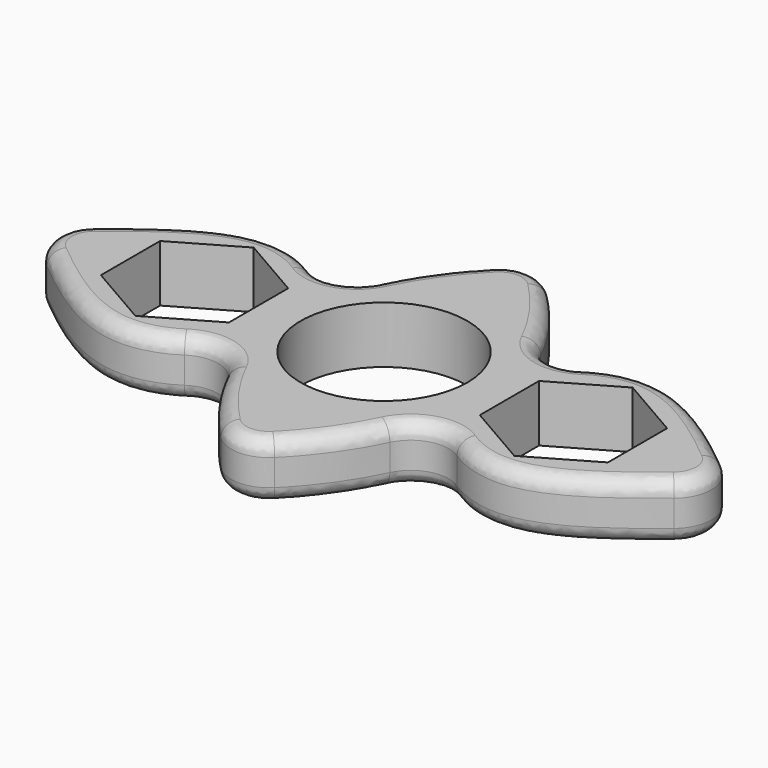
from build123d import *

# Parameters (mm, degrees)
F0_R     = 11
F1_DEPTH = 7.5
F2_R     = 5
F3_R     = 5
F4_R     = 2


# Not quite as in the source:
# - a feature names something its author has since deleted; it is built from what else it names


with BuildPart() as f1:
    # F0 (on Top) → F1 (new body)
    with BuildSketch(Plane.XY):
        with BuildLine():
            add(Edge.make_bspline(
                [(-13.295, 4.3866815476), (-12.5843159604, 8.4611271015), (-9.5128864845, 16.0598655207), (-3.7701811987, 22.6352872603), (0, 25.6154928356)],
                knots=[0, 0, 0, 0, 0.4861368513, 1, 1, 1, 1], degree=3))
            add(Edge.make_bspline(
                [(-13.295, 4.3866815476), (-14.8984951797, 9.3059969056), (-26.4777729526, 16.9391360967), (-38.4399958205, 6.3512038021), (-45.9589213133, 0)],
                knots=[0, 0, 0, 0, 0.4330873673, 1, 1, 1, 1], degree=3))
            add(Edge.make_bspline(
                [(-13.295, -4.3866815476), (-14.8984951797, -9.3059969056), (-26.4777729526, -16.9391360967), (-38.4399958205, -6.3512038021), (-45.9589213133, 0)],
                knots=[0, 0, 0, 0, 0.4330873673, 1, 1, 1, 1], degree=3))
            add(Edge.make_bspline(
                [(-13.295, -4.3866815476), (-12.5843159604, -8.4611271015), (-9.5128864845, -16.0598655207), (-3.7701811987, -22.6352872603), (0, -25.6154928356)],
                knots=[0, 0, 0, 0, 0.4861368513, 1, 1, 1, 1], degree=3))
            add(Edge.make_bspline(
                [(13.295, -4.3866815476), (12.5843159604, -8.4611271015), (9.5128864845, -16.0598655207), (3.7701811987, -22.6352872603), (0, -25.6154928356)],
                knots=[0, 0, 0, 0, 0.4861368513, 1, 1, 1, 1], degree=3))
            add(Edge.make_bspline(
                [(13.295, -4.3866815476), (14.8984951797, -9.3059969056), (26.4777729526, -16.9391360967), (38.4399958205, -6.3512038021), (45.9589213133, 0)],
                knots=[0, 0, 0, 0, 0.4330873673, 1, 1, 1, 1], degree=3))
            add(Edge.make_bspline(
                [(13.295, 4.3866815476), (14.8984951797, 9.3059969056), (26.4777729526, 16.9391360967), (38.4399958205, 6.3512038021), (45.9589213133, 0)],
                knots=[0, 0, 0, 0, 0.4330873673, 1, 1, 1, 1], degree=3))
            add(Edge.make_bspline(
                [(13.295, 4.3866815476), (12.5843159604, 8.4611271015), (9.5128864845, 16.0598655207), (3.7701811987, 22.6352872603), (0, 25.6154928356)],
                knots=[0, 0, 0, 0, 0.4861368513, 1, 1, 1, 1], degree=3))
        make_face()
        Polygon((-25, 9.7572195493), (-16.55, 4.8786097747), (-16.55, -4.8786097747), (-25, -9.7572195493), (-33.45, -4.8786097747), (-33.45, 4.8786097747), align=None, mode=Mode.SUBTRACT)
        Circle(F0_R, mode=Mode.SUBTRACT)
        Polygon((16.55, 4.8786097747), (25, 9.7572195493), (33.45, 4.8786097747), (33.45, -4.8786097747), (25, -9.7572195493), (16.55, -4.8786097747), align=None, mode=Mode.SUBTRACT)
    extrude(amount=F1_DEPTH)

    # F2
    f2_edges = [f1.edges().sort_by_distance(p)[0] for p in [
        (-13.295, -4.386682, 3.75),
        (13.295, -4.386682, 3.75),
        (13.295, 4.386682, 3.75),
        (-13.295, 4.386682, 3.75),
    ]]
    fillet(f2_edges, radius=F2_R)

    # F3
    f3_edges = [f1.edges().sort_by_distance(p)[0] for p in [
        (45.958921, 0, 3.75),
        (-45.958921, 0, 3.75),
        (0, 25.615493, 3.75),
        (0, -25.615493, 3.75),
    ]]
    fillet(f3_edges, radius=F3_R)

    # F4
    f4_edges = [f1.edges().sort_by_distance(p)[0] for p in [
        (-7.543737, 17.749498, 7.5),
        (-7.614373, 17.650431, 0),
        (0, 23.937425, 0),
        (-13.886715, 9.768638, 0),
        (7.614373, 17.650431, 0),
        (-29.206827, 11.687531, 0),
        (13.886715, 9.768638, 0),
        (-43.189272, 0, 0),
        (29.206827, 11.687531, 0),
        (-29.206827, -11.687531, 0),
        (43.189272, 0, 0),
        (-13.886715, -9.768638, 0),
        (29.206827, -11.687531, 0),
        (-7.614373, -17.650431, 0),
        (13.886715, -9.768638, 0),
        (0, -23.937425, 0),
        (7.614373, -17.650431, 0),
        (0, 23.937425, 7.5),
        (-13.886715, 9.768638, 7.5),
        (7.614373, 17.650431, 7.5),
        (-29.206827, 11.687531, 7.5),
        (13.886715, 9.768638, 7.5),
        (-43.189272, 0, 7.5),
        (29.206827, 11.687531, 7.5),
        (-29.206827, -11.687531, 7.5),
        (43.189272, 0, 7.5),
        (-13.886715, -9.768638, 7.5),
        (29.206827, -11.687531, 7.5),
        (-7.614373, -17.650431, 7.5),
        (13.886715, -9.768638, 7.5),
        (0, -23.937425, 7.5),
        (7.614373, -17.650431, 7.5),
    ]]
    fillet(f4_edges, radius=F4_R)


solid = f1.part
